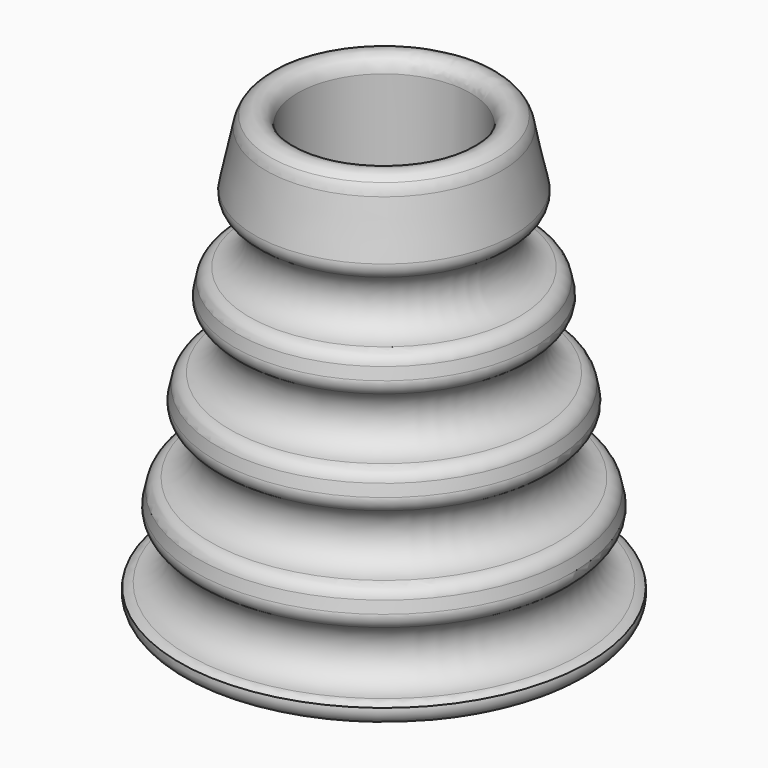
from build123d import *

# Parameters (mm, degrees)
F2_R = 0.5
F3_R = 1
F4_R = 0.5


# Not quite as in the source:
# - a fillet or chamfer that OpenCascade refuses, or shapes differently, is made with other operations: its cross-section is extruded or revolved along the edge and cut away or added


with BuildPart() as f1:
    # F0 (on Right) → F1 (revolve)
    with BuildSketch(Plane.YZ):
        with BuildLine():
            Line((1.6, 7), (1.6, 0))
            Line((1.6, 0), (7, 0))
            Line((7, 0), (6.8391733887, 0.7523472526))
            ThreePointArc((6.8391733887, 0.7523472526), (5.6465884719, 1.5199884269), (6.4210931851, 2.7081273941))
            Line((6.4210931851, 2.7081273941), (6.1745984239, 3.8612304467))
            ThreePointArc((6.1745984239, 3.8612304467), (4.9838910728, 4.6292824251), (5.7565143593, 5.81702865))
            Line((5.7565143593, 5.81702865), (5.5100226868, 6.9701172531))
            ThreePointArc((5.5100226868, 6.9701172531), (4.3211936737, 7.7385764233), (5.0919363056, 8.9259262934))
            Line((5.0919363056, 8.9259262934), (4.8454461776, 10.0790076719))
            ThreePointArc((4.8454461776, 10.0790076719), (3.6584962746, 10.8478704215), (4.4273590242, 12.0348203245))
            Line((4.4273590242, 12.0348203245), (3.7935030523, 15))
            Line((3.7935030523, 15), (2.9, 15))
            Line((2.9, 15), (2.9, 7))
            Line((2.9, 7), (1.6, 7))
        make_face()
    revolve(axis=Axis((0, 0, 4.2534018867), (0, 0, 1)))

    # F2
    f2_edges = [f1.edges().sort_by_distance(p)[0] for p in [
        (0, -7, 0),
    ]]
    fillet(f2_edges, radius=F2_R)

    # F3
    f3_edges = [f1.edges().sort_by_distance(p)[0] for p in [
        (0, -3.793503, 15),
    ]]
    fillet(f3_edges, radius=F3_R)

    # F4
    f4_edges = [f1.edges().sort_by_distance(p)[0] for p in [
        (0, -2.9, 15),
    ]]
    fillet(f4_edges, radius=F4_R)

    # F5: fillet of radius 0.5 on 8 edges, made by hand

    # F5_s1 → F5_t2 (revolve, cut)
    with BuildSketch(Plane.YZ):
        with BuildLine():
            ThreePointArc((6.3343268793, 3.1159338463), (6.3045099159, 2.812804601), (6.1047360241, 2.5828768236))
            Line((6.1047360241, 2.5828768236), (6.1308048817, 2.5400516514))
            ThreePointArc((6.1308048817, 2.5400516514), (6.275890142, 2.6126139907), (6.4312908518, 2.6590398365))
            Line((6.4312908518, 2.6590398365), (6.4701211283, 2.7186079241))
            ThreePointArc((6.4701211283, 2.7186079241), (6.4265423941, 2.9224693415), (6.3833548224, 3.1264143763))
            Line((6.3833548224, 3.1264143763), (6.3343268793, 3.1159338463))
        make_face()
    revolve(axis=Axis((0, 0, 2.7081273941), (0, 0, 1)), mode=Mode.SUBTRACT)

    # F5_s3 → F5_t4 (revolve, cut)
    with BuildSketch(Plane.YZ):
        with BuildLine():
            ThreePointArc((5.8352123602, 3.8467734878), (6.1111091916, 3.7184731822), (6.2620048701, 3.4542563694))
            Line((6.2620048701, 3.4542563694), (6.3110331203, 3.464736965))
            ThreePointArc((6.3110331203, 3.464736965), (6.2671343159, 3.6681821949), (6.223626674, 3.8717110423))
            Line((6.223626674, 3.8717110423), (6.1639294451, 3.910218048))
            ThreePointArc((6.1639294451, 3.910218048), (6.0033563992, 3.8893715312), (5.8415613594, 3.8965057953))
            Line((5.8415613594, 3.8965057953), (5.8352123602, 3.8467734878))
        make_face()
    revolve(axis=Axis((0, 0, 3.8612304467), (0, 0, 1)), mode=Mode.SUBTRACT)

    # F5_s5 → F5_t6 (revolve, cut)
    with BuildSketch(Plane.YZ):
        with BuildLine():
            ThreePointArc((5.6698902381, 6.2241699621), (5.6402076686, 5.9213515759), (5.4408793774, 5.6914640766))
            Line((5.4408793774, 5.6914640766), (5.4670065415, 5.6486740837))
            ThreePointArc((5.4670065415, 5.6486740837), (5.6117441038, 5.721334738), (5.7668064169, 5.7679604755))
            Line((5.7668064169, 5.7679604755), (5.8055426094, 5.8275092456))
            ThreePointArc((5.8055426094, 5.8275092456), (5.7620349676, 6.031038093), (5.7189184882, 6.2346505578))
            Line((5.7189184882, 6.2346505578), (5.6698902381, 6.2241699621))
        make_face()
    revolve(axis=Axis((0, 0, 5.81702865), (0, 0, 1)), mode=Mode.SUBTRACT)

    # F5_s7 → F5_t8 (revolve, cut)
    with BuildSketch(Plane.YZ):
        with BuildLine():
            ThreePointArc((5.1711676686, 6.9562404165), (5.4466411354, 6.8277953589), (5.5972871086, 6.5638075666))
            Line((5.5972871086, 6.5638075666), (5.6463156669, 6.5742882281))
            ThreePointArc((5.6463156669, 6.5742882281), (5.6024878748, 6.7774012627), (5.5590512451, 6.9805979146))
            Line((5.5590512451, 6.9805979146), (5.4994478138, 7.0191255774))
            ThreePointArc((5.4994478138, 7.0191255774), (5.3391021848, 6.9985989442), (5.1775842829, 7.005964363))
            Line((5.1775842829, 7.005964363), (5.1711676686, 6.9562404165))
        make_face()
    revolve(axis=Axis((0, 0, 6.9701172531), (0, 0, 1)), mode=Mode.SUBTRACT)

    # F5_s9 → F5_t10 (revolve, cut)
    with BuildSketch(Plane.YZ):
        with BuildLine():
            ThreePointArc((5.0054542089, 9.3324032148), (4.9759058858, 9.0298959251), (4.7770231397, 8.8000494176))
            Line((4.7770231397, 8.8000494176), (4.803208591, 8.7572946993))
            ThreePointArc((4.803208591, 8.7572946993), (4.9475987292, 8.8300529979), (5.1023227169, 8.8768776823))
            Line((5.1023227169, 8.8768776823), (5.1409648639, 8.9364069549))
            ThreePointArc((5.1409648639, 8.9364069549), (5.0975282343, 9.1396036069), (5.0544827672, 9.3428838763))
            Line((5.0544827672, 9.3428838763), (5.0054542089, 9.3324032148))
        make_face()
    revolve(axis=Axis((0, 0, 8.9259262934), (0, 0, 1)), mode=Mode.SUBTRACT)

    # F5_s11 → F5_t12 (revolve, cut)
    with BuildSketch(Plane.YZ):
        with BuildLine():
            ThreePointArc((4.5071225679, 10.06570926), (4.7821724292, 9.9371201252), (4.9325687342, 9.6733616312))
            Line((4.9325687342, 9.6733616312), (4.9815976017, 9.6838423588))
            ThreePointArc((4.9815976017, 9.6838423588), (4.9378407422, 9.8866235704), (4.8944750452, 10.0894883995))
            Line((4.8944750452, 10.0894883995), (4.83496545, 10.1280365395))
            ThreePointArc((4.83496545, 10.1280365395), (4.6748475582, 10.1078289), (4.5136068189, 10.1154247505))
            Line((4.5136068189, 10.1154247505), (4.5071225679, 10.06570926))
        make_face()
    revolve(axis=Axis((0, 0, 10.0790076719), (0, 0, 1)), mode=Mode.SUBTRACT)

    # F5_s13 → F5_t14 (revolve, cut)
    with BuildSketch(Plane.YZ):
        with BuildLine():
            ThreePointArc((4.3410187927, 12.4406336001), (4.3116045686, 12.1384376452), (4.1131673115, 11.9086328438))
            Line((4.1131673115, 11.9086328438), (4.139411031, 11.8659134958))
            ThreePointArc((4.139411031, 11.8659134958), (4.2834540181, 11.9387687688), (4.4378397518, 11.985791457))
            Line((4.4378397518, 11.985791457), (4.4763878918, 12.0453010521))
            ThreePointArc((4.4763878918, 12.0453010521), (4.4330221948, 12.2481658812), (4.3900476603, 12.4511143277))
            Line((4.3900476603, 12.4511143277), (4.3410187927, 12.4406336001))
        make_face()
    revolve(axis=Axis((0, 0, 12.0348203245), (0, 0, 1)), mode=Mode.SUBTRACT)

    # F5_s15 → F5_t16 (revolve, cut)
    with BuildSketch(Plane.YZ):
        with BuildLine():
            ThreePointArc((6.8710397119, 0.6048203506), (6.7294416847, 0.6937195092), (6.5664861101, 0.7311166003))
            Line((6.5664861101, 0.7311166003), (6.5693955756, 0.7811677314))
            ThreePointArc((6.5693955756, 0.7811677314), (6.6996233982, 0.7821433999), (6.8284103438, 0.8013139513))
            Line((6.8284103438, 0.8013139513), (6.8882013319, 0.7628277826))
            ThreePointArc((6.8882013319, 0.7628277826), (6.9039766947, 0.6890305995), (6.9044045376, 0.6422418567))
            Line((6.9044045376, 0.6422418567), (6.8710397119, 0.6048203506))
        make_face()
    revolve(axis=Axis((0, 0, 0.7523472526), (0, 0, 1)), mode=Mode.SUBTRACT)


solid = f1.part
